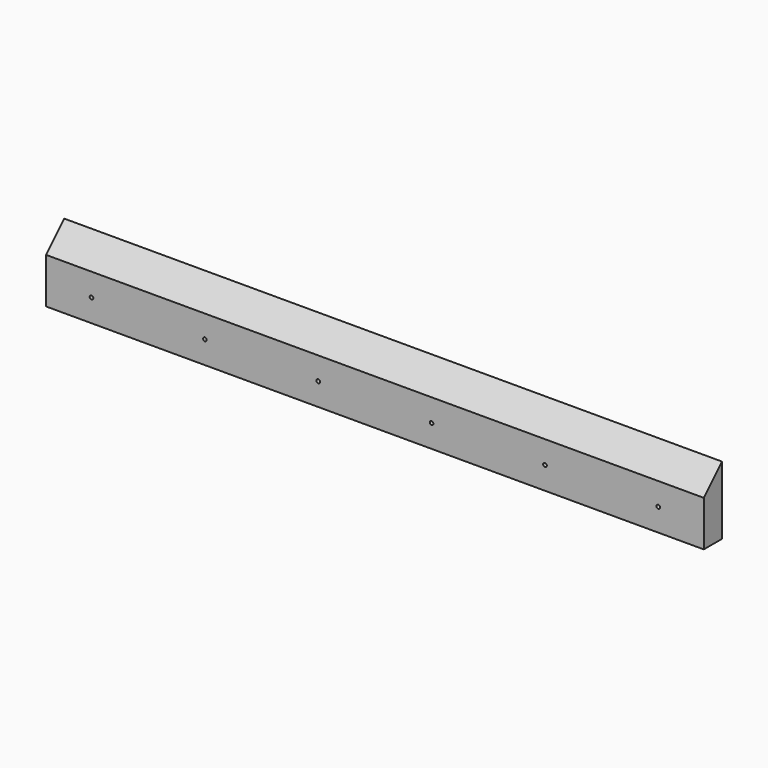
from build123d import *

# Parameters (mm, degrees)
F4_W           = 25
F4_H           = 75
F0_DEPTH       = 724
F1_SIZE        = 24.99999
F3_D           = 4
F3_CSINK_D     = 10
F3_CSINK_ANGLE = 90


# Not quite as in the source:
# - a fillet or chamfer is up to 0.001 mm smaller than in the source, because OpenCascade refuses the exact size
# - a feature names something its author has since deleted; it is built from what else it names


with BuildPart() as f0:
    # F4 (on Right) → F0 (new body)
    with BuildSketch(Plane.YZ):
        Rectangle(F4_W, F4_H)
    extrude(amount=F0_DEPTH)

    # F1 (size 25 in the source; OpenCascade refuses exactly that, so slightly less here)
    f1_edges = [f0.edges().sort_by_distance(p)[0] for p in [
        (362, -12.5, 37.5),
    ]]
    chamfer(f1_edges, length=F1_SIZE)

    # F3 (through all)
    with Locations(Plane(origin=(0, 12.5, 0), x_dir=(-1, 0, 0), z_dir=(0, 1, 0))):
        with Locations((-50, -12.5), (-174.8, -12.5), (-299.6, -12.5), (-424.4, -12.5), (-549.2, -12.5), (-674, -12.5)):
            CounterSinkHole(F3_D / 2, F3_CSINK_D / 2, counter_sink_angle=F3_CSINK_ANGLE)


solid = f0.part
